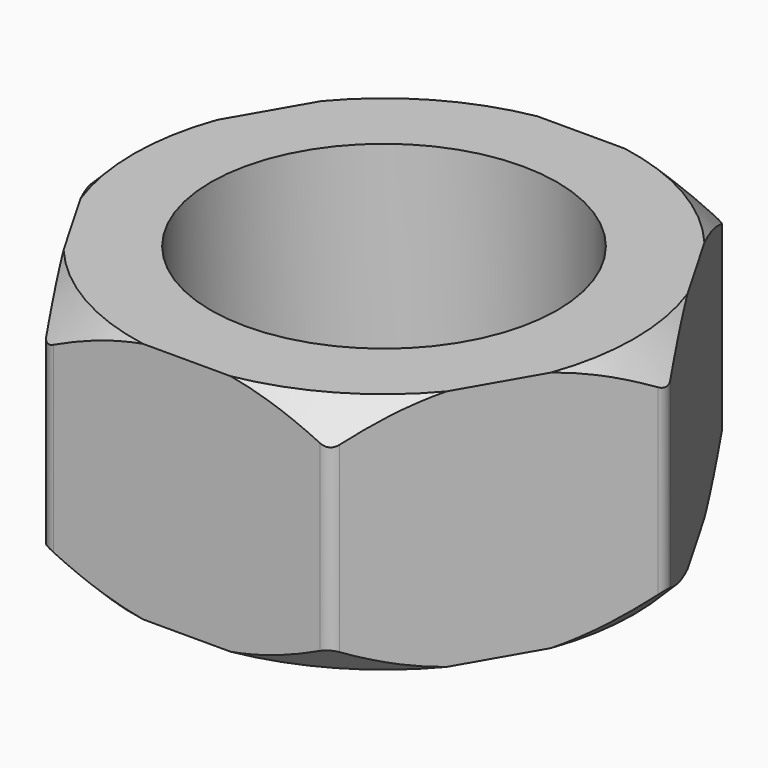
from build123d import *

# Parameters (mm, degrees)
F1_DEPTH = 6.3
F2_R     = 0.4
F5_D     = 9


with BuildPart() as f1:
    # F0 (on Top) → F1 (new body)
    with BuildSketch(Plane.XY):
        Polygon((7.3900834456, 0), (3.6950417228, 6.4), (-3.6950417228, 6.4), (-7.3900834456, 0), (-3.6950417228, -6.4), (3.6950417228, -6.4), align=None)
    extrude(amount=F1_DEPTH)

    # F2
    f2_edges = [f1.edges().sort_by_distance(p)[0] for p in [
        (-3.695042, -6.4, 3.15),
        (3.695042, -6.4, 3.15),
        (7.390083, 0, 3.15),
        (3.695042, 6.4, 3.15),
        (-3.695042, 6.4, 3.15),
        (-7.390083, 0, 3.15),
    ]]
    fillet(f2_edges, radius=F2_R)

    # F3 (on Right) → F4 (revolve, cut)
    with BuildSketch(Plane.YZ):
        Polygon((9.5, 6.3), (6.5, 6.3), (9.5, 3.3), align=None)
        Polygon((9.5, 3), (6.5, 0), (9.5, 0), align=None)
    revolve(axis=Axis((0, 0, 10.4480586015), (0, 0, -1)), mode=Mode.SUBTRACT)

    # F5 (through all)
    with Locations(Plane(origin=(0, 0, 0), x_dir=(1, 0, 0), z_dir=(0, 0, -1))):
        with Locations((0, 0)):
            Hole(F5_D / 2)


solid = f1.part
